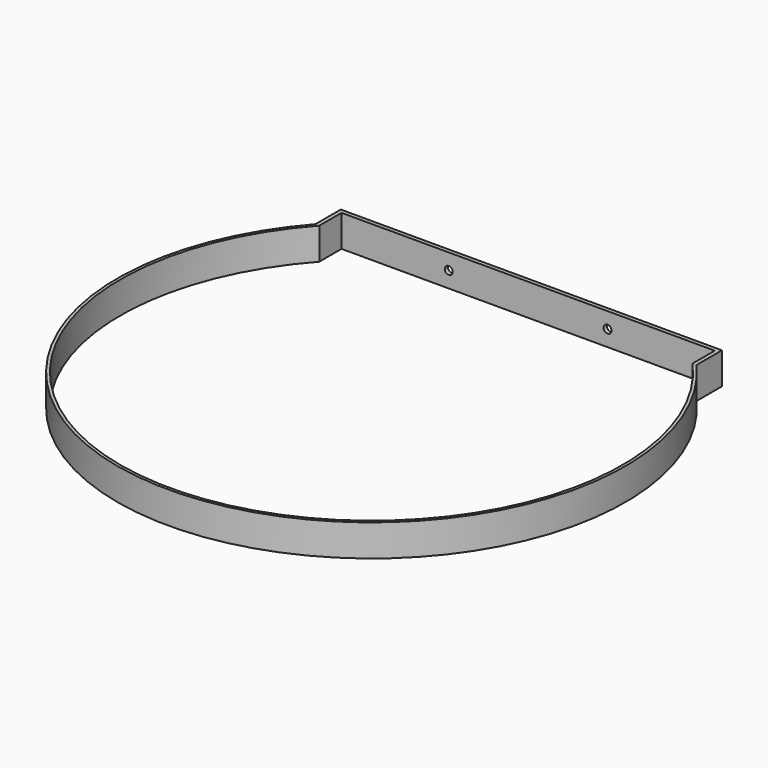
from build123d import *

# Parameters (mm, degrees)
F1_DEPTH = 25.4
F3_DEPTH = 25.4
F5_DEPTH = 363.0051666021


with BuildPart() as f1:
    # F0 (on Top) → F1 (new body)
    with BuildSketch(Plane.XY):
        Polygon((152.4, 0), (-152.4, 0), (-152.4, -25.4), (-149.225, -25.4), (-149.225, -3.175), (149.225, -3.175), (149.225, -25.4), (152.4, -25.4), align=None)
    extrude(amount=F1_DEPTH)

    # F4 (on face) → F5 (cut, through all)
    with BuildSketch(Plane(origin=(0, 0, 0), x_dir=(-1, 0, 0), z_dir=(0, 1, 0))):
        with BuildLine():
            ThreePointArc((-60.325, 12.7), (-63.5, 15.875), (-66.675, 12.7))
            Line((-66.675, 12.7), (-60.325, 12.7))
        make_face()
        with BuildLine():
            ThreePointArc((66.675, 12.7), (63.5, 15.875), (60.325, 12.7))
            Line((60.325, 12.7), (66.675, 12.7))
        make_face()
        with BuildLine():
            Line((66.675, 12.7), (60.325, 12.7))
            ThreePointArc((60.325, 12.7), (63.5, 9.525), (66.675, 12.7))
        make_face()
        with BuildLine():
            Line((-60.325, 12.7), (-66.675, 12.7))
            ThreePointArc((-66.675, 12.7), (-63.5, 9.525), (-60.325, 12.7))
        make_face()
    extrude(amount=-F5_DEPTH, mode=Mode.SUBTRACT)


with BuildPart() as f3:
    # F2 (on face) → F3 (new body)
    with BuildSketch(Plane.XY.offset(25.4)):
        with BuildLine():
            Line((-149.225, -25.4), (-152.4, -25.4))
            ThreePointArc((-152.4, -25.4), (0, -363.0041666021), (152.4, -25.4))
            Line((152.4, -25.4), (149.225, -25.4))
            ThreePointArc((149.225, -25.4), (0, -360.6338970331), (-149.225, -25.4))
        make_face()
    extrude(amount=-F3_DEPTH)


solid = Compound([f1.part, f3.part])
